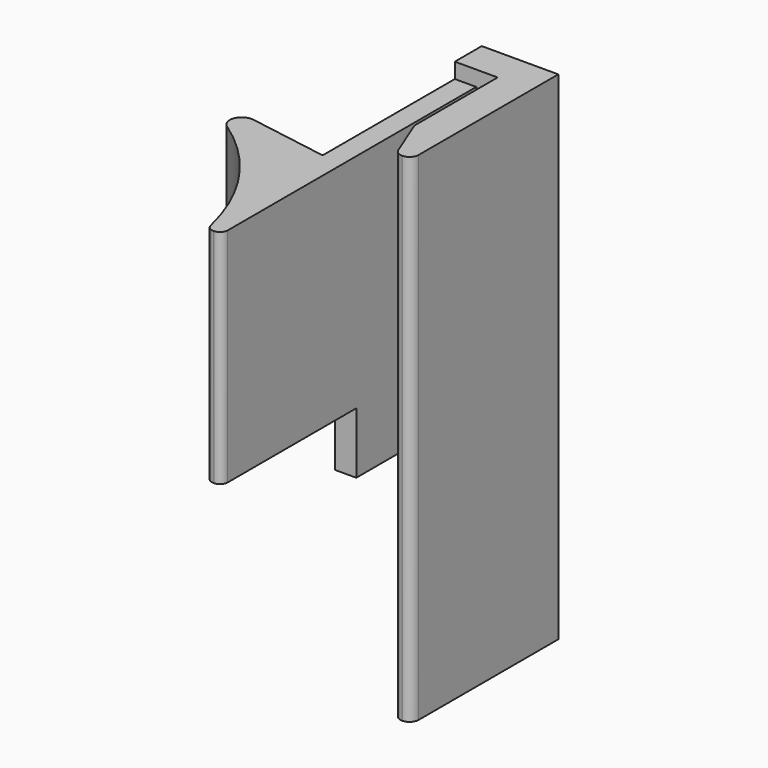
from build123d import *

# Parameters (mm, degrees)
F0_W     = 1.4
F0_H     = 9.8
F1_DEPTH = 15.5
F2_DEPTH = 19.5
F3_DEPTH = 1
F4_DEPTH = 32.5


# Not quite as in the source:
# - ends of sketch curves that miss each other by under 0.0002 mm in the source are joined


with BuildPart() as f1:
    # F0 (on Top) → F1 (new body)
    with BuildSketch(Plane.XY):
        with BuildLine():
            Line((-32.0736061335, 18.2974073312), (-37.0736061335, 18.2974073312))
            Line((-37.0736061335, 18.2974073312), (-37.0736061335, 16.0974073312))
            Line((-37.0736061335, 16.0974073312), (-35.6736061335, 16.0974073312))
            Line((-35.6736061335, 16.0974073312), (-34.2736061335, 16.0974073312))
            Line((-34.2736061335, 16.0974073312), (-34.2736061335, 9.4129567733))
            ThreePointArc((-34.2736061335, 9.4129567733), (-34.2627799655, 9.2994922606), (-34.230692148, 9.1901223675))
            Line((-34.230692148, 9.1901223675), (-33.2244723711, 6.6745729254))
            ThreePointArc((-33.2244723711, 6.6745729254), (-33.0063342171, 6.402317089), (-32.6736057993, 6.2974395666))
            Line((-32.6736057993, 6.2974395666), (-32.6673863566, 6.2974073312))
            ThreePointArc((-32.6673863566, 6.2974073312), (-32.2471488287, 6.4753478956), (-32.0736061335, 6.8974073312))
            Line((-32.0736061335, 6.8974073312), (-32.0736061335, 18.2974073312))
        make_face()
        with Locations((-36.3736061335, 11.1974073312)):
            Rectangle(F0_W, F0_H)
        with BuildLine():
            Line((-35.6736061335, 6.2974073312), (-37.0736061335, 6.2974073312))
            Line((-37.0736061335, 6.2974073312), (-37.0736061335, 5.2974073312))
            Line((-37.0736061335, 5.2974073312), (-42.2844909944, 6.1658881413))
            ThreePointArc((-42.2844909944, 6.1658881413), (-42.8770439673, 6.0305679631), (-43.2034719774, 5.5178542706))
            ThreePointArc((-43.2034719774, 5.5178542706), (-43.1469979089, 5.0781395288), (-42.8650641349, 4.7360113048))
            ThreePointArc((-42.8650641349, 4.7360113048), (-38.9420533833, 0.8088724995), (-36.7058590055, -4.271665588))
            ThreePointArc((-36.7058590055, -4.271665588), (-36.5388782387, -4.5797772785), (-36.2106530565, -4.7025926688))
            Line((-36.2106530565, -4.7025926688), (-36.1736061335, -4.7025926688))
            ThreePointArc((-36.1736061335, -4.7025926688), (-35.8200527429, -4.5561460594), (-35.6736061335, -4.2025926688))
            Line((-35.6736061335, -4.2025926688), (-35.6736061335, 6.2974073312))
        make_face()
    extrude(amount=-F1_DEPTH)

    # F0 (on Top) → F2 (join)
    with BuildSketch(Plane.XY):
        with Locations((-36.3736061335, 11.1974073312)):
            Rectangle(F0_W, F0_H)
    extrude(amount=-F2_DEPTH)

    # F0 (on Top) → F3 (cut)
    with BuildSketch(Plane.XY):
        with Locations((-36.3736061335, 11.1974073312)):
            Rectangle(F0_W, F0_H)
        with BuildLine():
            Line((-35.6736061335, 6.2974073312), (-37.0736061335, 6.2974073312))
            Line((-37.0736061335, 6.2974073312), (-37.0736061335, 5.2974073312))
            Line((-37.0736061335, 5.2974073312), (-42.2844909944, 6.1658881413))
            ThreePointArc((-42.2844909944, 6.1658881413), (-42.8770439673, 6.0305679631), (-43.2034719774, 5.5178542706))
            ThreePointArc((-43.2034719774, 5.5178542706), (-43.1469979089, 5.0781395288), (-42.8650641349, 4.7360113048))
            ThreePointArc((-42.8650641349, 4.7360113048), (-38.9420533833, 0.8088724995), (-36.7058590055, -4.271665588))
            ThreePointArc((-36.7058590055, -4.271665588), (-36.5388782387, -4.5797772785), (-36.2106530565, -4.7025926688))
            Line((-36.2106530565, -4.7025926688), (-36.1736061335, -4.7025926688))
            ThreePointArc((-36.1736061335, -4.7025926688), (-35.8200527429, -4.5561460594), (-35.6736061335, -4.2025926688))
            Line((-35.6736061335, -4.2025926688), (-35.6736061335, 6.2974073312))
        make_face()
    extrude(amount=-F3_DEPTH, mode=Mode.SUBTRACT)

    # F0 (on Top) → F4 (join)
    with BuildSketch(Plane.XY):
        with BuildLine():
            Line((-32.0736061335, 18.2974073312), (-37.0736061335, 18.2974073312))
            Line((-37.0736061335, 18.2974073312), (-37.0736061335, 16.0974073312))
            Line((-37.0736061335, 16.0974073312), (-35.6736061335, 16.0974073312))
            Line((-35.6736061335, 16.0974073312), (-34.2736061335, 16.0974073312))
            Line((-34.2736061335, 16.0974073312), (-34.2736061335, 9.4129567733))
            ThreePointArc((-34.2736061335, 9.4129567733), (-34.2627799655, 9.2994922606), (-34.230692148, 9.1901223675))
            Line((-34.230692148, 9.1901223675), (-33.2244723711, 6.6745729254))
            ThreePointArc((-33.2244723711, 6.6745729254), (-33.0063342171, 6.402317089), (-32.6736057993, 6.2974395666))
            Line((-32.6736057993, 6.2974395666), (-32.6673863566, 6.2974073312))
            ThreePointArc((-32.6673863566, 6.2974073312), (-32.2471488287, 6.4753478956), (-32.0736061335, 6.8974073312))
            Line((-32.0736061335, 6.8974073312), (-32.0736061335, 18.2974073312))
        make_face()
    extrude(amount=-F4_DEPTH)


solid = f1.part
